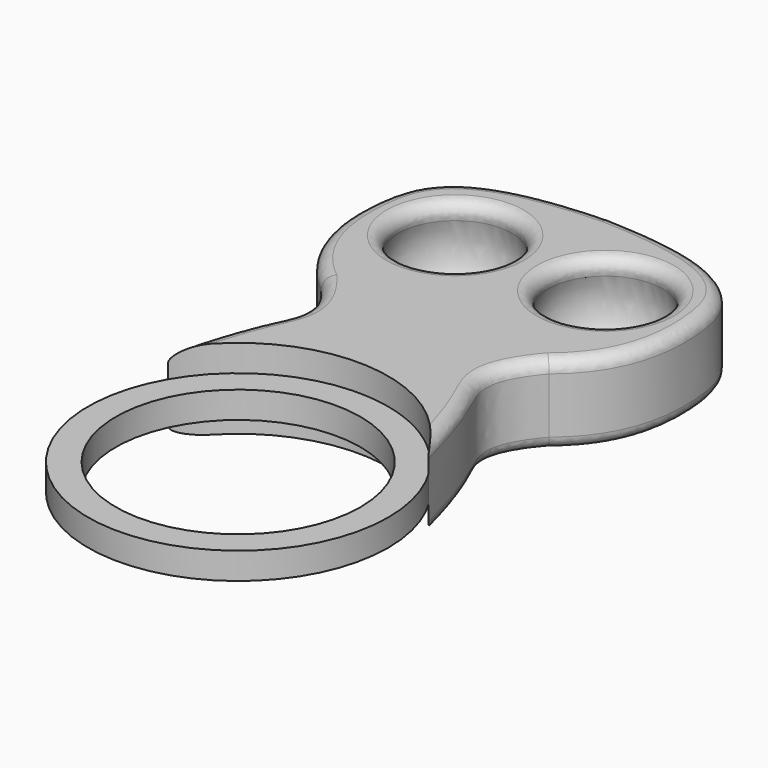
from build123d import *

# Parameters (mm, degrees)
F0_R     = 5.55
F3_DEPTH = 7.2
F7_R     = 1.1
F2_R     = 13.5
F2_R_2   = 11
F8_DEPTH = 2.4
F9_R     = 1.1


with BuildPart() as f3:
    # F0 (on Top) → F3 (new body)
    with BuildSketch(Plane.XY):
        with BuildLine():
            ThreePointArc((-11.6930940819, 6.7505532951), (-0.0017511308, 13.5005532951), (11.6895918203, 6.7505532951))
            add(Edge.make_bspline(
                [(11.6895918203, 6.7505532951), (9.9671929403, 13.2683368526), (8.461780314, 15.2310629248), (7.581869113, 19.0145089795), (10.2478263318, 22.1374873967)],
                knots=[0, 0, 0, 0, 0.5531001172, 1, 1, 1, 1], degree=3))
            add(Edge.make_bspline(
                [(10.2478263318, 22.1374873967), (14.2370524614, 25.3879677824), (15.7755501979, 34.5383314318), (12.4803592801, 41.667265907), (-0.0017511308, 42.0005532951)],
                knots=[0, 0, 0, 0, 0.4566129243, 1, 1, 1, 1], degree=3))
            add(Edge.make_bspline(
                [(-10.2513285935, 22.1374873967), (-14.2405547231, 25.3879677824), (-15.7790524596, 34.5383314318), (-12.4838615418, 41.667265907), (-0.0017511308, 42.0005532951)],
                knots=[0, 0, 0, 0, 0.4566129243, 1, 1, 1, 1], degree=3))
            add(Edge.make_bspline(
                [(-11.6930940819, 6.7505532951), (-9.970695202, 13.2683368526), (-8.4652825756, 15.2310629248), (-7.5853713746, 19.0145089795), (-10.2513285935, 22.1374873967)],
                knots=[0, 0, 0, 0, 0.5531001172, 1, 1, 1, 1], degree=3))
        make_face()
        with Locations((-6.7517511308, 32.823843971)):
            Circle(F0_R, mode=Mode.SUBTRACT)
        with Locations((6.7482488692, 32.823843971)):
            Circle(F0_R, mode=Mode.SUBTRACT)
        with Locations((-6.7517511308, 32.823843971)):
            Circle(F0_R)
        with Locations((6.7482488692, 32.823843971)):
            Circle(F0_R)
    extrude(amount=F3_DEPTH)

    # F5 (on offset) → F6 (revolve, cut)
    with BuildSketch(Plane.XY.offset(3.6)):
        with BuildLine():
            Line((-12.3017511308, 32.823843971), (-1.2017511308, 32.823843971))
            ThreePointArc((-1.2017511308, 32.823843971), (-6.7517511308, 38.373843971), (-12.3017511308, 32.823843971))
        make_face()
        with BuildLine():
            ThreePointArc((12.2982488692, 32.823843971), (6.7482488692, 38.373843971), (1.1982488692, 32.823843971))
            Line((1.1982488692, 32.823843971), (12.2982488692, 32.823843971))
        make_face()
    revolve(axis=Axis((-6.7517511308, 32.823843971, 3.6), (1, 0, 0)), mode=Mode.SUBTRACT)

    # F7
    f7_edges = [f3.edges().sort_by_distance(p)[0] for p in [
        (-6.751751, 37.047882, 7.2),
        (6.748249, 37.047882, 7.2),
    ]]
    fillet(f7_edges, radius=F7_R)

    # F9
    f9_edges = [f3.edges().sort_by_distance(p)[0] for p in [
        (-9.097493, 14.612429, 7.2),
        (-9.097493, 14.612429, 0),
        (9.093991, 14.612429, 0),
        (9.093991, 14.612429, 7.2),
        (13.952844, 36.5096, 7.2),
        (-13.956346, 36.5096, 7.2),
        (-13.956346, 36.5096, 0),
        (13.952844, 36.5096, 0),
    ]]
    fillet(f9_edges, radius=F9_R)


with BuildPart() as f8:
    # F2 (on offset) → F8 (new body)
    with BuildSketch(Plane.XY.offset(2.4)):
        with Locations((-0.0017511308, 0.0005532951)):
            Circle(F2_R)
        with Locations((-0.0017511308, 0.0005532951)):
            Circle(F2_R_2, mode=Mode.SUBTRACT)
    extrude(amount=F8_DEPTH)


solid = Compound([f3.part, f8.part])
